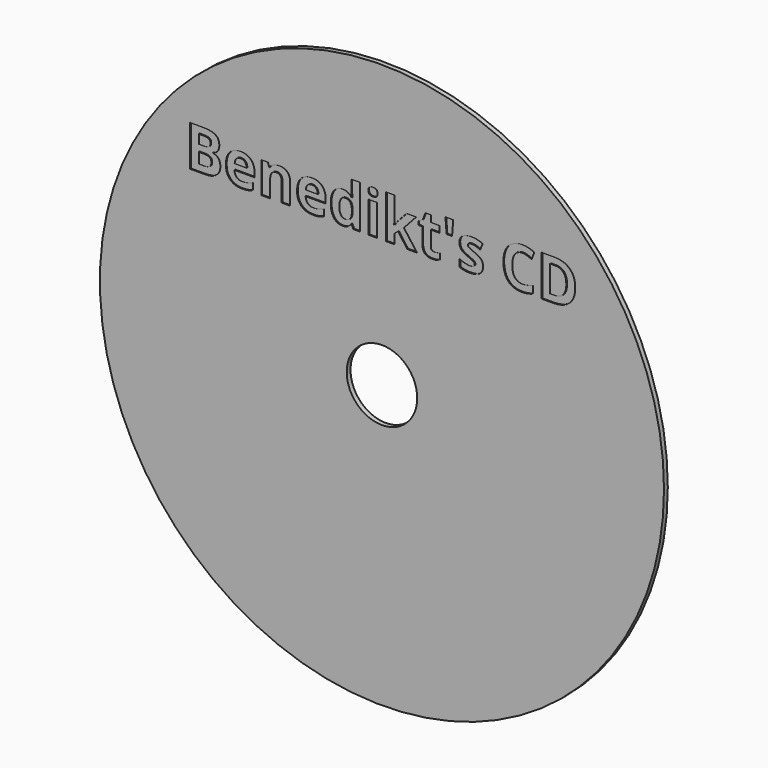
from build123d import *

# Parameters (mm, degrees)
F0_R         = 60
F0_R_2       = 7.5
F1_DEPTH     = 1.01
F2_TEXT_SIZE = 12.1269349216
F3_DEPTH     = 0.2


# Not quite as in the source:
# - Text() gives the source's letters only with a copy of the font that has no kerning and outlines rounded to 1/6400 em; it was checked with that copy


with BuildPart() as f1:
    # F0 (on Front) → F1 (new body)
    with BuildSketch(Plane.XZ):
        Circle(F0_R)
        Circle(F0_R_2, mode=Mode.SUBTRACT)
    extrude(amount=F1_DEPTH)

    # F2 (on face) → F3 (cut)
    with BuildSketch(Plane.XZ.offset(1.01)):
        with Locations((-41.8899357319, 27.2207483649)):
            Text("Benedikt's CD", F2_TEXT_SIZE, font='Open Sans', font_style=FontStyle.BOLD, text_align=(TextAlign.LEFT, TextAlign.BOTTOM))
    extrude(amount=-F3_DEPTH, mode=Mode.SUBTRACT)


solid = f1.part
